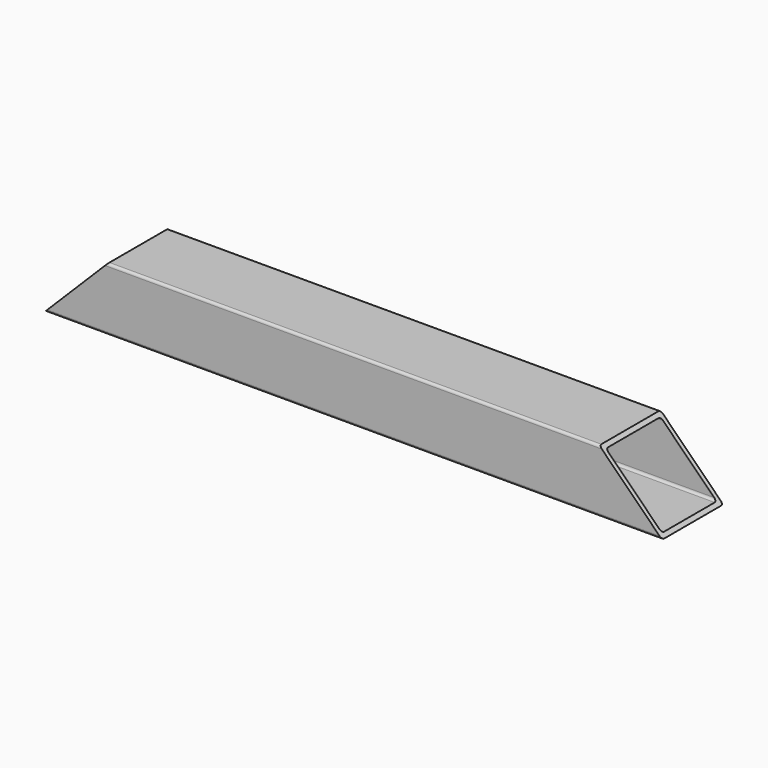
from build123d import *

# Parameters (mm, degrees)
F0_W     = 157.2524309158
F0_H     = 129.0383934975
F0_W_2   = 140.655875206
F0_H_2   = 115.3461933136
F1_DEPTH = 635
F2_R     = 5.08
F4_DEPTH = 157.2534309158


# Not quite as in the source:
# - a pattern or mirror of a feature is missing from the dataset's text; its kind, count and spacing are read off the source's solid


with BuildPart() as f1:
    # F0 (on Right) → F1 (new body, symmetric)
    with BuildSketch(Plane.YZ):
        Rectangle(F0_W, F0_H)
        Rectangle(F0_W_2, F0_H_2, mode=Mode.SUBTRACT)
    extrude(amount=F1_DEPTH, both=True)

    # F2
    f2_edges = [f1.edges().sort_by_distance(p)[0] for p in [
        (0, -78.626215, 64.519197),
        (0, -70.327938, 57.673097),
        (0, 70.327938, 57.673097),
        (0, 78.626215, 64.519197),
        (0, 78.626215, -64.519197),
        (0, 70.327938, -57.673097),
        (0, -70.327938, -57.673097),
        (0, -78.626215, -64.519197),
    ]]
    fillet(f2_edges, radius=F2_R)

    # F3 (on face) → F4 (cut, through all)
    with BuildSketch(Plane.XZ.offset(78.6262154579)):
        Polygon((635, -64.5191967487), (635, 64.5191967487), (505.9616065025, 64.5191967487), align=None)
    f4 = extrude(amount=-F4_DEPTH, mode=Mode.SUBTRACT)

    # F4_copies: F4 across plane
    add(f4.mirror(Plane(origin=(0, 0, 0), x_dir=(0, 0, -1), z_dir=(-1, 0, 0))), mode=Mode.SUBTRACT)


solid = f1.part
